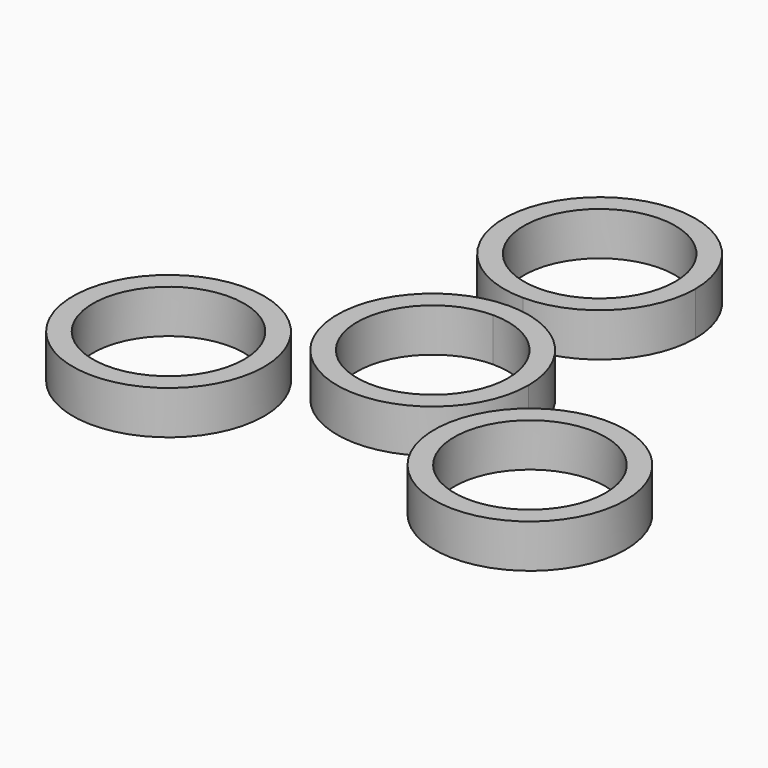
from build123d import *

# Parameters (mm, degrees)
F1_DEPTH = 6.35
F0_R     = 13.97
F0_R_2   = 11.049


with BuildPart() as f1:
    # F0 (on Top) → F1 (new body)
    with BuildSketch(Plane.XY):
        with BuildLine():
            ThreePointArc((13.97, 30.48), (-9.8782817332, 40.3582817332), (0, 16.51))
            ThreePointArc((0, 16.51), (9.8782817332, 20.6017182668), (13.97, 30.48))
        make_face()
        with BuildLine():
            ThreePointArc((11.049, 30.48), (7.8128228253, 22.6671771747), (0, 19.431))
            ThreePointArc((0, 19.431), (-7.8128228253, 38.2928228253), (11.049, 30.48))
        make_face(mode=Mode.SUBTRACT)
    extrude(amount=F1_DEPTH)


with BuildPart() as f1b:
    # F0 (on Top) → F1, piece 2 (new body)
    with BuildSketch(Plane.XY):
        with Locations((26.3964543073, -15.24)):
            Circle(F0_R)
        with Locations((26.3964543073, -15.24)):
            Circle(F0_R_2, mode=Mode.SUBTRACT)
    extrude(amount=F1_DEPTH)


with BuildPart() as f1c:
    # F0 (on Top) → F1, piece 3 (new body)
    with BuildSketch(Plane.XY):
        with Locations((-26.3964543073, -15.24)):
            Circle(F0_R)
        with Locations((-26.3964543073, -15.24)):
            Circle(F0_R_2, mode=Mode.SUBTRACT)
    extrude(amount=F1_DEPTH)


with BuildPart() as f1d:
    # F0 (on Top) → F1, piece 4 (new body)
    with BuildSketch(Plane.XY):
        with BuildLine():
            ThreePointArc((13.97, 0), (9.8782817332, 9.8782817332), (0, 13.97))
            ThreePointArc((0, 13.97), (-9.8782817332, -9.8782817332), (13.97, 0))
        make_face()
        with BuildLine():
            ThreePointArc((0, 11.049), (7.8128228253, 7.8128228253), (11.049, 0))
            ThreePointArc((11.049, 0), (-7.8128228253, -7.8128228253), (0, 11.049))
        make_face(mode=Mode.SUBTRACT)
    extrude(amount=F1_DEPTH)


solid = Compound([f1.part, f1b.part, f1c.part, f1d.part])
